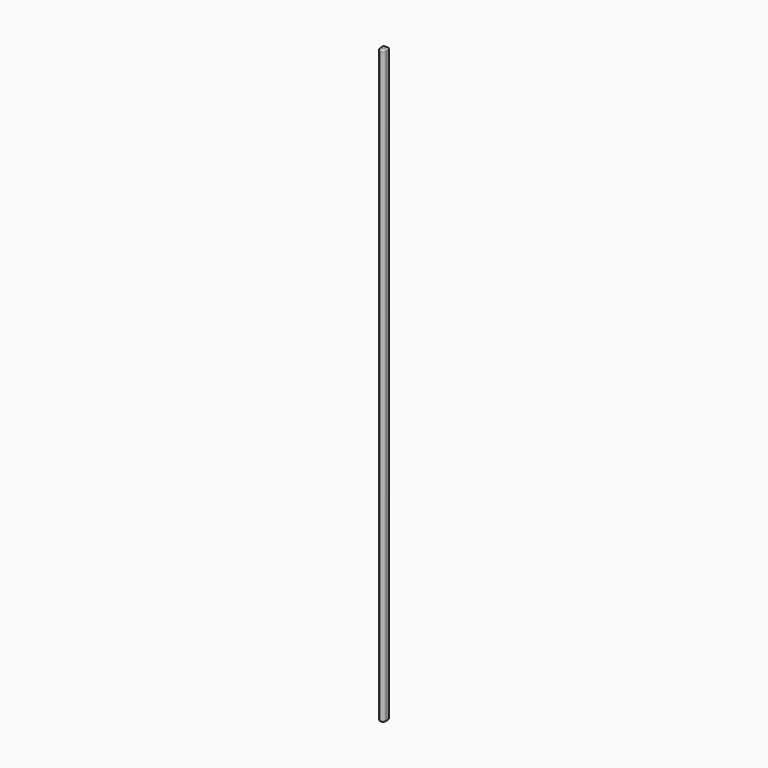
from build123d import *

# Parameters (mm, degrees)
F0_W     = 12.7
F0_H     = 15.875
F1_DEPTH = 609.6
F2_R     = 3.175
F3_R     = 6.34999
F4_R     = 3.175
F6_D     = 3.571875
F6_DEPTH = 9.525
F6_TIP   = 1.0730995118


# Not quite as in the source:
# - a fillet or chamfer is up to 0.001 mm smaller than in the source, because OpenCascade refuses the exact size


with BuildPart() as f1:
    # F0 (on Top) → F1 (new body, symmetric)
    with BuildSketch(Plane.XY):
        Rectangle(F0_W, F0_H)
    extrude(amount=F1_DEPTH, both=True)

    # F2
    f2_edges = [f1.edges().sort_by_distance(p)[0] for p in [
        (6.35, 7.9375, 0),
        (-6.35, 7.9375, 0),
    ]]
    fillet(f2_edges, radius=F2_R)

    # F3 (radius 6.35 in the source; OpenCascade refuses exactly that, so slightly less here)
    f3_edges = [f1.edges().sort_by_distance(p)[0] for p in [
        (-6.35, -7.9375, 0),
        (6.35, -7.9375, 0),
    ]]
    fillet(f3_edges, radius=F3_R)

    # F4
    f4_edges = [f1.edges().sort_by_distance(p)[0] for p in [
        (6.35, 1.587495, 609.6),
        (4.490131, -6.077631, 609.6),
        (5.420064, 7.007564, 609.6),
        (0, -7.9375, 609.6),
        (0, 7.9375, 609.6),
        (-4.490131, -6.077631, 609.6),
        (-5.420064, 7.007564, 609.6),
        (-6.35, 1.587495, 609.6),
        (6.35, 1.587495, -609.6),
        (4.490131, -6.077631, -609.6),
        (5.420064, 7.007564, -609.6),
        (0, -7.9375, -609.6),
        (0, 7.9375, -609.6),
        (-4.490131, -6.077631, -609.6),
        (-5.420064, 7.007564, -609.6),
        (-6.35, 1.587495, -609.6),
    ]]
    fillet(f4_edges, radius=F4_R)

    # F6
    with Locations(Plane(origin=(0, 7.9375, 0), x_dir=(-1, 0, 0), z_dir=(0, 1, 0))):
        with Locations((0, 558.8), (0, 476.25), (0, 393.7), (0, 311.15), (0, 228.6), (0, 146.05), (0, 63.5), (0, -19.05), (0, -101.6), (0, -184.15), (0, -266.7), (0, -349.25), (0, -431.8), (0, -514.35)):
            Hole(F6_D / 2, depth=F6_DEPTH)
            with Locations((0, 0, -(F6_DEPTH + F6_TIP / 2))):  # 118° drill point
                Cone(0, F6_D / 2, F6_TIP, mode=Mode.SUBTRACT)


solid = f1.part
